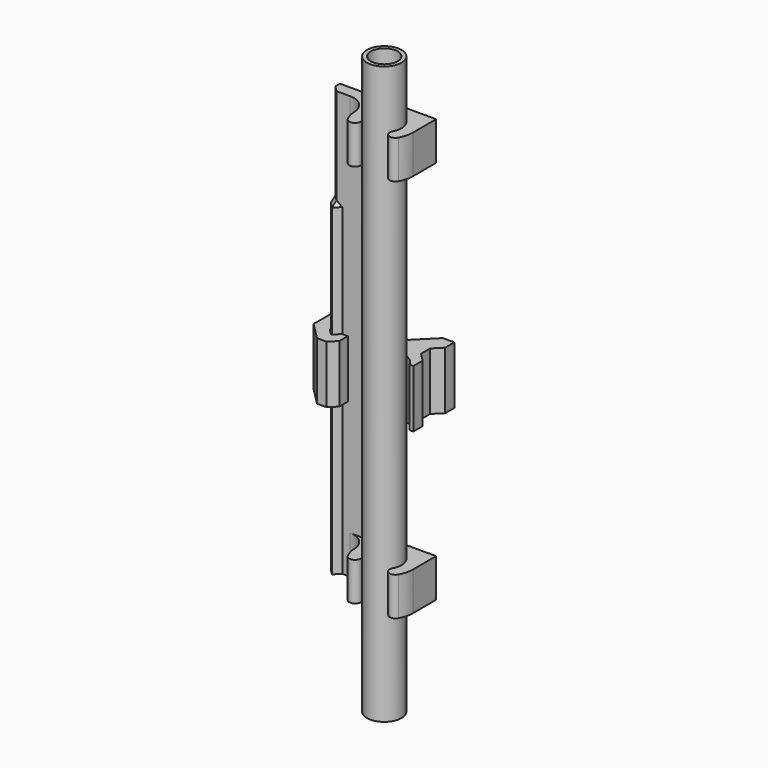
from build123d import *

# Parameters (mm, degrees)
F3_DEPTH      = 10
F4_START      = -100
F4_DEPTH      = 10
F5_DEPTH      = 110
F6_DEPTH      = 85
F7_T1_DEPTH   = 10
F7_T3_DEPTH   = 10
F1_R          = 4.5
F1_R_2        = 3.5
F8_DEPTH      = 125
F8_DEPTH_BACK = 25
F9_START      = 40
F9_DEPTH      = 15
F10_SIZE      = 1.5
F11_SIZE      = 1.05


# Not quite as in the source:
# - a fillet or chamfer that OpenCascade refuses, or shapes differently, is made with other operations: its cross-section is extruded or revolved along the edge and cut away or added
# - a feature names something its author has since deleted; it is built from what else it names


with BuildPart() as f3:
    # F0 (on Top) → F3 (new body)
    with BuildSketch(Plane.XY):
        Polygon((-14.5, 4.5), (-7.5, 4.5), (-5, 7), (-5, 7.5), (-17.5, 7.5), (-17.5, 4.5), align=None)
        with BuildLine():
            ThreePointArc((-7.5, 0), (-7.2618437741, -1.875), (-6.5625, -3.6309218871))
            ThreePointArc((-6.5625, -3.6309218871), (-4.5238156226, -4.2172375097), (-3.9375, -2.1785531322))
            ThreePointArc((-3.9375, -2.1785531322), (0, 4.5), (3.9375, -2.1785531322))
            ThreePointArc((3.9375, -2.1785531322), (4.5238156226, -4.2172375097), (6.5625, -3.6309218871))
            ThreePointArc((6.5625, -3.6309218871), (7.2618437741, -1.875), (7.5, 0))
            Line((7.5, 0), (7.5, 7.5))
            Line((7.5, 7.5), (-5, 7.5))
            Line((-5, 7.5), (-5, 7))
            Line((-5, 7), (-7.5, 4.5))
            Line((-7.5, 4.5), (-7.5, 0))
        make_face()
    extrude(amount=F3_DEPTH)



with BuildPart() as f4:
    # F3_face (on face) → F4 (new body)
    with BuildSketch(Plane(origin=(-2.7583074733, 3.5975142137, 0), x_dir=(1, 0, 0), z_dir=(0, 0, -1)).offset(F4_START)):
        with BuildLine():
            Line((-14.7416925267, -3.9024857863), (10.2583074733, -3.9024857863))
            Line((10.2583074733, -3.9024857863), (10.2583074733, 3.5975142137))
            ThreePointArc((10.2583074733, 3.5975142137), (10.0201512474, 5.4725142137), (9.3208074733, 7.2284361007))
            ThreePointArc((9.3208074733, 7.2284361007), (7.2821230959, 7.8147517233), (6.6958074733, 5.7760673459))
            ThreePointArc((6.6958074733, 5.7760673459), (2.7583074733, -0.9024857863), (-1.1791925267, 5.7760673459))
            ThreePointArc((-1.1791925267, 5.7760673459), (-1.7655081493, 7.8147517233), (-3.8041925267, 7.2284361007))
            ThreePointArc((-3.8041925267, 7.2284361007), (-4.5035363009, 5.4725142137), (-4.7416925267, 3.5975142137))
            Line((-4.7416925267, 3.5975142137), (-4.7416925267, -0.9024857863))
            Line((-4.7416925267, -0.9024857863), (-14.7416925267, -0.9024857863))
            Line((-14.7416925267, -0.9024857863), (-14.7416925267, -3.9024857863))
        make_face()
    extrude(amount=-F4_DEPTH)


with BuildPart() as f3_1:
    add(f3.part)

    add(f4.part)  # F5 merges F4
    # F0 (on Top) → F5 (join, through all)
    with BuildSketch(Plane.XY):
        Polygon((-14.5, 4.5), (-7.5, 4.5), (-5, 7), (-5, 7.5), (-17.5, 7.5), (-17.5, 4.5), align=None)
    extrude(amount=F5_DEPTH)

    # F0 (on Top) → F6 (join)
    with BuildSketch(Plane.XY):
        Polygon((-16, 3), (-14.5, 4.5), (-17.5, 4.5), align=None)
    extrude(amount=F6_DEPTH)

    # F7: fillet of radius 5 on 2 edges, made by hand

    # F7_s2 → F7_t1 (join)
    with BuildSketch(Plane.XY):
        with BuildLine():
            ThreePointArc((-12.4899959968, 4.5), (-9.0258943817, 3.1055512755), (-7.4939975981, -0.3))
            Line((-7.4939975981, -0.3), (-6.9943977582, -0.28))
            ThreePointArc((-6.9943977582, -0.28), (-7, 0), (-7, 4.5))
            Line((-7, 4.5), (-7.5, 5))
            Line((-7.5, 5), (-12.4899959968, 5))
            Line((-12.4899959968, 5), (-12.4899959968, 4.5))
        make_face()
    extrude(amount=F7_T1_DEPTH)

    # F7_s4 → F7_t3 (join)
    with BuildSketch(Plane.XY.offset(100)):
        with BuildLine():
            ThreePointArc((-7.4939975981, -0.3), (-9.0258943817, 3.1055512755), (-12.4899959968, 4.5))
            Line((-12.4899959968, 4.5), (-12.4899959968, 5))
            Line((-12.4899959968, 5), (-7.5, 5))
            Line((-7.5, 5), (-7, 4.5))
            ThreePointArc((-7, 4.5), (-7, 0), (-6.9943977582, -0.28))
            Line((-6.9943977582, -0.28), (-7.4939975981, -0.3))
        make_face()
    extrude(amount=F7_T3_DEPTH)

    # F10
    f10_edges = [f3_1.edges().sort_by_distance(p)[0] for p in [
        (-17.5, 4.5, 97.5),
    ]]
    chamfer(f10_edges, length=F10_SIZE)

    # F11
    f11_edges = [f3_1.edges().sort_by_distance(p)[0] for p in [
        (-16.75, 3.75, 85),
        (-15.25, 3.75, 85),
    ]]
    chamfer(f11_edges, length=F11_SIZE)


with BuildPart() as f8:
    # F1 (on Top) → F8 (new body, two sides)
    with BuildSketch(Plane.XY) as f8_sk:
        Circle(F1_R)
        Circle(F1_R_2, mode=Mode.SUBTRACT)
    extrude(amount=F8_DEPTH)
    extrude(f8_sk.sketch, amount=-F8_DEPTH_BACK)


with BuildPart() as f9:
    # F2 (on Top) → F9 (new body)
    with BuildSketch(Plane.XY.offset(F9_START)):
        with BuildLine():
            Line((-16, 2.7171572875), (-17.7, 4.4171572875))
            Line((-17.7, 4.4171572875), (-17.7, 7.7))
            Line((-17.7, 7.7), (-4.8, 7.7))
            Line((-4.8, 7.7), (-4.8, 6.9171572875))
            Line((-4.8, 6.9171572875), (-5.6816604165, 6.035496871))
            Line((-5.6816604165, 6.035496871), (-5.6816604165, 2.375827381))
            Line((-5.6816604165, 2.375827381), (-4.6816604165, 2.375827381))
            ThreePointArc((-4.6816604165, 2.375827381), (0, 5.25), (4.6816604165, 2.375827381))
            Line((4.6816604165, 2.375827381), (5.6816604165, 2.375827381))
            Line((5.6816604165, 2.375827381), (5.6816604165, 5.375827381))
            Line((5.6816604165, 5.375827381), (3.519574107, 7.5379136905))
            Line((3.519574107, 7.5379136905), (3.519574107, 10.5379136905))
            Line((3.519574107, 10.5379136905), (5.6816604165, 12.7))
            Line((5.6816604165, 12.7), (5.6816604165, 15.7))
            Line((5.6816604165, 15.7), (2.6816604165, 15.7))
            Line((2.6816604165, 15.7), (-2.3183395835, 10.7))
            Line((-2.3183395835, 10.7), (-13.7, 10.7))
            Line((-13.7, 10.7), (-18.7, 15.7))
            Line((-18.7, 15.7), (-21.7, 15.7))
            Line((-21.7, 15.7), (-21.7, 4.1745166004))
            Line((-21.7, 4.1745166004), (-17.2426406871, -0.2828427125))
            Line((-17.2426406871, -0.2828427125), (-14.7573593129, -0.2828427125))
            Line((-14.7573593129, -0.2828427125), (-12.9171572875, 1.5573593129))
            Line((-12.9171572875, 1.5573593129), (-12.9171572875, 4.3))
            Line((-12.9171572875, 4.3), (-14.4171572875, 4.3))
            Line((-14.4171572875, 4.3), (-16, 2.7171572875))
        make_face()
    extrude(amount=F9_DEPTH)


solid = Compound([f3_1.part, f8.part, f9.part])
